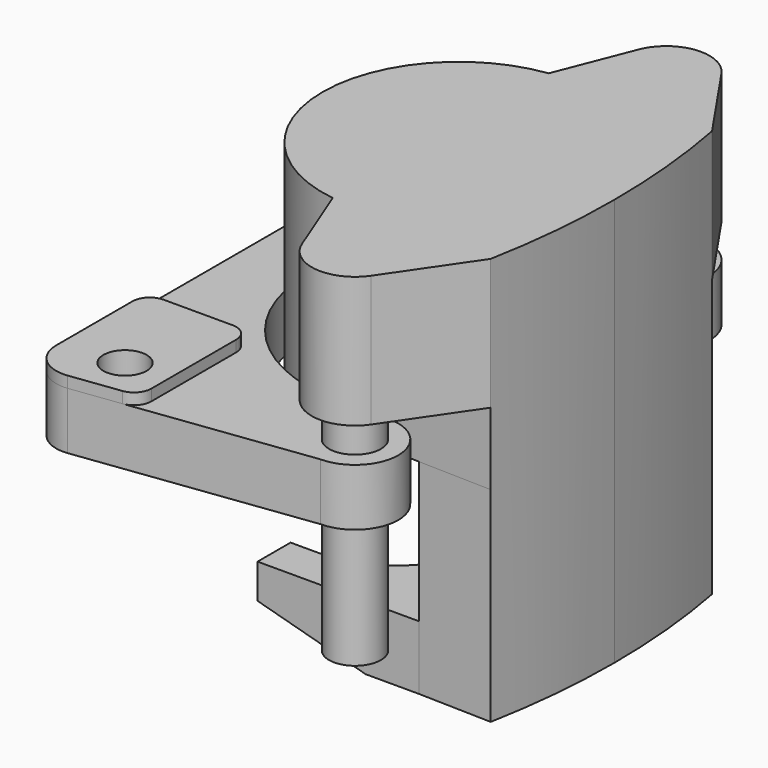
from build123d import *

# Parameters (mm, degrees)
F1_DEPTH  = 13.2
F2_R      = 8
F4_DEPTH  = 2.6
F5_R      = 5
F6_DEPTH  = 15.801
F7_R      = 6
F8_DEPTH  = 25
F10_START = 4.5
F9_R      = 31.5
F10_DEPTH = 47
F12_DEPTH = 30.3
F13_R     = 19.5
F14_DEPTH = 25
F15_R     = 6
F16_DEPTH = 51
F18_DEPTH = 16.7
F20_DEPTH = 64
F22_DEPTH = 14.8
F24_DEPTH = 93.444683


with BuildPart() as f1:
    # F0 (on Top) → F1 (new body)
    with BuildSketch(Plane.XY):
        with BuildLine():
            Line((-41.036294, 63), (-41.036294, 0))
            Line((-41.036294, 0), (-41.036294, -63))
            Line((-41.036294, -63), (20.963706, -55))
            ThreePointArc((20.963706, -55), (30.963706, -45), (20.963706, -35))
            Line((20.963706, -35), (8.963706, -35))
            ThreePointArc((8.963706, -35), (-15.785031, -24.748737), (-26.036294, 0))
            ThreePointArc((-26.036294, 0), (-15.785031, 24.748737), (8.963706, 35))
            Line((8.963706, 35), (20.963706, 35))
            ThreePointArc((20.963706, 35), (30.963706, 45), (20.963706, 55))
            Line((20.963706, 55), (-41.036294, 63))
        make_face()
    extrude(amount=F1_DEPTH)

    # F2
    f2_edges = [f1.edges().sort_by_distance(p)[0] for p in [
        (-41.036294, -63, 6.6),
        (-41.036294, 63, 6.6),
    ]]
    fillet(f2_edges, radius=F2_R)

    # F3 (on face) → F4 (join)
    with BuildSketch(Plane.XY.offset(13.2)):
        with BuildLine():
            ThreePointArc((-32.012523, 61.835642), (-38.318805, 59.909338), (-41.036294, 53.90142))
            Line((-41.036294, 53.90142), (-41.036294, 31.835642))
            ThreePointArc((-41.036294, 31.835642), (-39.864721, 29.007215), (-37.036294, 27.835642))
            Line((-37.036294, 27.835642), (-21.036294, 27.835642))
            ThreePointArc((-21.036294, 27.835642), (-18.207867, 29.007215), (-17.036294, 31.835642))
            Line((-17.036294, 31.835642), (-17.036294, 56.386194))
            ThreePointArc((-17.036294, 56.386194), (-18.032335, 59.027449), (-20.524409, 60.353305))
            Line((-20.524409, 60.353305), (-32.012523, 61.835642))
        make_face()
        with BuildLine():
            Line((-32.012523, -61.835642), (-20.524409, -60.353305))
            ThreePointArc((-20.524409, -60.353305), (-18.032335, -59.027449), (-17.036294, -56.386194))
            Line((-17.036294, -56.386194), (-17.036294, -31.835642))
            ThreePointArc((-17.036294, -31.835642), (-18.207867, -29.007215), (-21.036294, -27.835642))
            Line((-21.036294, -27.835642), (-37.036294, -27.835642))
            ThreePointArc((-37.036294, -27.835642), (-39.864721, -29.007215), (-41.036294, -31.835642))
            Line((-41.036294, -31.835642), (-41.036294, -53.90142))
            ThreePointArc((-41.036294, -53.90142), (-38.318805, -59.909338), (-32.012523, -61.835642))
        make_face()
    extrude(amount=F4_DEPTH)

    # F5 (on face) → F6 (cut, through all)
    with BuildSketch(Plane.XY.offset(15.8)):
        with Locations((-27.036294, 51.5)):
            Circle(F5_R)
        with Locations((-27.036294, -51.5)):
            Circle(F5_R)
    extrude(amount=-F6_DEPTH, mode=Mode.SUBTRACT)

    # F7 (on face) → F8 (cut)
    with BuildSketch(Plane.XY.offset(13.2)):
        with Locations((20.963706, 45)):
            Circle(F7_R)
        with Locations((20.963706, -45)):
            Circle(F7_R)
    extrude(amount=-F8_DEPTH, mode=Mode.SUBTRACT)


with BuildPart() as f10:
    # F9 (on Top) → F10 (new body)
    with BuildSketch(Plane.XY.offset(F10_START)):
        with Locations((8.963706, 0)):
            Circle(F9_R)
    extrude(amount=F10_DEPTH)

    # F11 (on face) → F12 (join, through all)
    with BuildSketch(Plane.XY.offset(51.5)):
        with BuildLine():
            ThreePointArc((29.219138, -50.64339), (30.517614, -47.953446), (30.963706, -45))
            ThreePointArc((30.963706, -45), (19.100639, -35.175084), (11.65791, -48.660896))
            ThreePointArc((11.65791, -48.660896), (19.841928, -54.936881), (29.219138, -50.64339))
        make_face()
        with BuildLine():
            ThreePointArc((11.65791, -48.660896), (19.100639, -35.175084), (30.963706, -45))
            ThreePointArc((30.963706, -45), (30.517614, -47.953446), (29.219138, -50.64339))
            Line((29.219138, -50.64339), (41.963706, -32))
            ThreePointArc((41.963706, -32), (44.212065, -16.070159), (44.963706, 0))
            ThreePointArc((44.963706, 0), (44.212065, 16.070159), (41.963706, 32))
            Line((41.963706, 32), (29.219138, 50.64339))
            ThreePointArc((29.219138, 50.64339), (30.517614, 47.953446), (30.963706, 45))
            ThreePointArc((30.963706, 45), (19.100639, 35.175084), (11.65791, 48.660896))
            Line((11.65791, 48.660896), (4.797982, 31.223337))
            Line((4.797982, 31.223337), (4.797982, 0))
            Line((4.797982, 0), (4.797982, -31.223337))
            Line((4.797982, -31.223337), (11.65791, -48.660896))
        make_face()
        with BuildLine():
            ThreePointArc((29.219138, 50.64339), (19.841928, 54.936881), (11.65791, 48.660896))
            ThreePointArc((11.65791, 48.660896), (19.100639, 35.175084), (30.963706, 45))
            ThreePointArc((30.963706, 45), (30.517614, 47.953446), (29.219138, 50.64339))
        make_face()
    extrude(amount=-F12_DEPTH)

    # F13 (on face) → F14 (cut)
    with BuildSketch(Plane(origin=(0, 0, 4.5), x_dir=(1, 0, 0), z_dir=(0, 0, -1))):
        with Locations((8.963706, 0)):
            Circle(F13_R)
    extrude(amount=-F14_DEPTH, mode=Mode.SUBTRACT)

    # F15 (on face) → F16 (join)
    with BuildSketch(Plane(origin=(0, 0, 21.2), x_dir=(1, 0, 0), z_dir=(0, 0, -1))):
        with Locations((20.963706, -45)):
            Circle(F15_R)
        with Locations((20.963706, 45)):
            Circle(F15_R)
    extrude(amount=F16_DEPTH)

    # F17 (on face) → F18 (join, through all)
    with BuildSketch(Plane(origin=(0, 0, 21.2), x_dir=(1, 0, 0), z_dir=(0, 0, -1))):
        with BuildLine():
            Line((13.12943, -31.223337), (41.963706, -32))
            ThreePointArc((41.963706, -32), (44.212065, -16.070159), (44.963706, 0))
            ThreePointArc((44.963706, 0), (44.212065, 16.070159), (41.963706, 32))
            Line((41.963706, 32), (13.12943, 31.223337))
            Line((13.12943, 31.223337), (32.089781, 0))
            Line((32.089781, 0), (13.12943, -31.223337))
        make_face()
    extrude(amount=F18_DEPTH)

    # F19 (on face) → F20 (join)
    with BuildSketch(Plane(origin=(0, 0, 21.2), x_dir=(1, 0, 0), z_dir=(0, 0, -1))):
        with BuildLine():
            Line((24.969869, -31.542264), (41.963706, -32))
            ThreePointArc((41.963706, -32), (44.212065, -16.070159), (44.963706, 0))
            ThreePointArc((44.963706, 0), (44.212065, 16.070159), (41.963706, 32))
            Line((41.963706, 32), (24.969869, 31.542264))
            Line((24.969869, 31.542264), (24.969869, -31.542264))
        make_face()
    extrude(amount=F20_DEPTH)

    # F21 (on face) → F22 (join, through all)
    with BuildSketch(Plane(origin=(0, 0, -42.8), x_dir=(1, 0, 0), z_dir=(0, 0, -1))):
        with BuildLine():
            Line((24.969869, 0), (24.969869, 31.542264))
            Line((24.969869, 31.542264), (-12.340831, 31.542264))
            Line((-12.340831, 31.542264), (-12.340831, 22))
            Line((-12.340831, 22), (-5.585416, 22))
            ThreePointArc((-5.585416, 22), (9.970933, 15.556349), (16.414584, 0))
            ThreePointArc((16.414584, 0), (9.970933, -15.556349), (-5.585416, -22))
            Line((-5.585416, -22), (-12.340831, -22))
            Line((-12.340831, -22), (-12.340831, -31.542264))
            Line((-12.340831, -31.542264), (24.969869, -31.542264))
            Line((24.969869, -31.542264), (24.969869, 0))
        make_face()
    extrude(amount=-F22_DEPTH)

    # F23 (on face) → F24 (cut, through all)
    with BuildSketch(Plane(origin=(0, 31.542264, 0), x_dir=(-1, 0, 0), z_dir=(0, 1, 0))):
        Polygon((12.340831, -42.8), (12.340831, -36), (-12.659169, -42.8), align=None)
    extrude(amount=-F24_DEPTH, mode=Mode.SUBTRACT)


solid = Compound([f1.part, f10.part])
